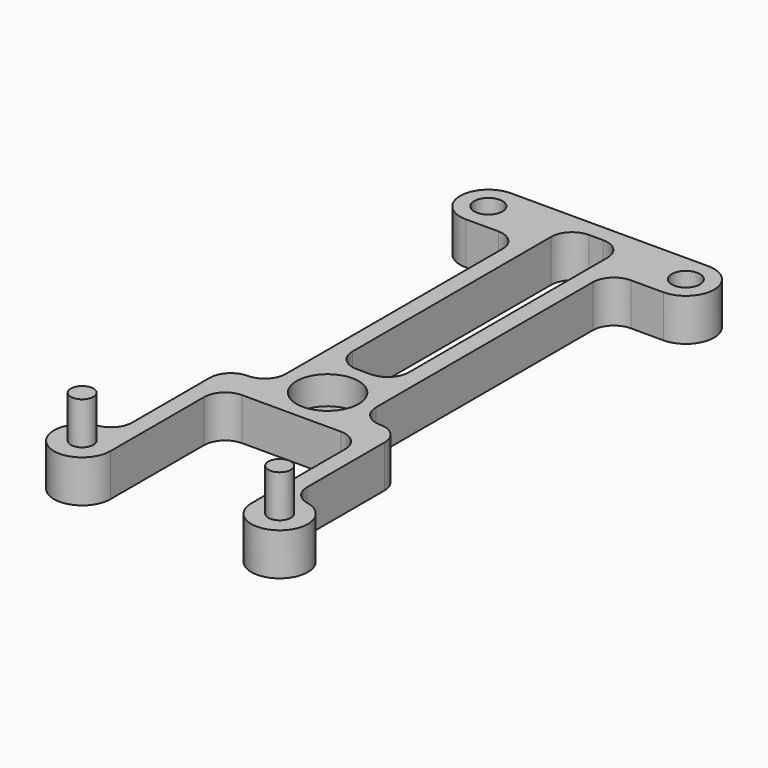
from build123d import *

# Parameters (mm, degrees)
F0_R     = 1.524
F0_R_2   = 1.27
F0_W     = 5.08
F0_H     = 26.162
F1_DEPTH = 3.81
F2_R     = 1.90499
F3_R     = 1.016
F4_DEPTH = 3.81
F5_R     = 2.794
F6_DEPTH = 2.54


# Not quite as in the source:
# - a fillet or chamfer is up to 0.001 mm smaller than in the source, because OpenCascade refuses the exact size


with BuildPart() as f1:
    # F0 (on Top) → F1 (new body)
    with BuildSketch(Plane.XY):
        with BuildLine():
            ThreePointArc((-8.89, 31.75), (-11.43, 29.21), (-8.89, 26.67))
            Line((-8.89, 26.67), (-4.064, 26.67))
            Line((-4.064, 26.67), (-4.064, -1.524))
            Line((-4.064, -1.524), (-7.874, -1.524))
            Line((-7.874, -1.524), (-7.874, -13.97))
            Line((-7.874, -13.97), (-8.89, -13.97))
            ThreePointArc((-8.89, -13.97), (-10.6860512242, -18.3060512242), (-6.35, -16.51))
            Line((-6.35, -16.51), (-6.35, -4.064))
            Line((-6.35, -4.064), (6.35, -4.064))
            Line((6.35, -4.064), (6.35, -16.51))
            ThreePointArc((6.35, -16.51), (10.6860512242, -18.3060512242), (8.89, -13.97))
            Line((8.89, -13.97), (7.874, -13.97))
            Line((7.874, -13.97), (7.874, -1.524))
            Line((7.874, -1.524), (4.064, -1.524))
            Line((4.064, -1.524), (4.064, 26.67))
            Line((4.064, 26.67), (8.89, 26.67))
            ThreePointArc((8.89, 26.67), (11.43, 29.21), (8.89, 31.75))
            Line((8.89, 31.75), (-8.89, 31.75))
        make_face()
        Circle(F0_R, mode=Mode.SUBTRACT)
        with Locations((-8.89, 29.21)):
            Circle(F0_R_2, mode=Mode.SUBTRACT)
        with Locations((0, 17.145)):
            Rectangle(F0_W, F0_H, mode=Mode.SUBTRACT)
        with Locations((8.89, 29.21)):
            Circle(F0_R_2, mode=Mode.SUBTRACT)
    extrude(amount=F1_DEPTH)

    # F2 (radius 1.905 in the source; OpenCascade refuses exactly that, so slightly less here)
    f2_edges = [f1.edges().sort_by_distance(p)[0] for p in [
        (6.35, -4.064, 1.905),
        (-6.35, -4.064, 1.905),
        (-4.064, -1.524, 1.905),
        (-7.874, -1.524, 1.905),
        (7.874, -1.524, 1.905),
        (4.064, 26.67, 1.905),
        (4.064, -1.524, 1.905),
        (-4.064, 26.67, 1.905),
        (2.54, 30.226, 1.905),
        (-2.54, 30.226, 1.905),
        (-2.54, 4.064, 1.905),
        (2.54, 4.064, 1.905),
        (7.874, -13.97, 1.905),
        (-7.874, -13.97, 1.905),
    ]]
    fillet(f2_edges, radius=F2_R)

    # F3 (on face) → F4 (join)
    with BuildSketch(Plane.XY.offset(3.81)):
        with Locations((-8.89, -16.51)):
            Circle(F3_R)
        with Locations((8.89, -16.51)):
            Circle(F3_R)
    extrude(amount=F4_DEPTH)

    # F5 (on face) → F6 (cut)
    with BuildSketch(Plane.XY.offset(3.81)):
        Circle(F5_R)
    extrude(amount=-F6_DEPTH, mode=Mode.SUBTRACT)


solid = f1.part
